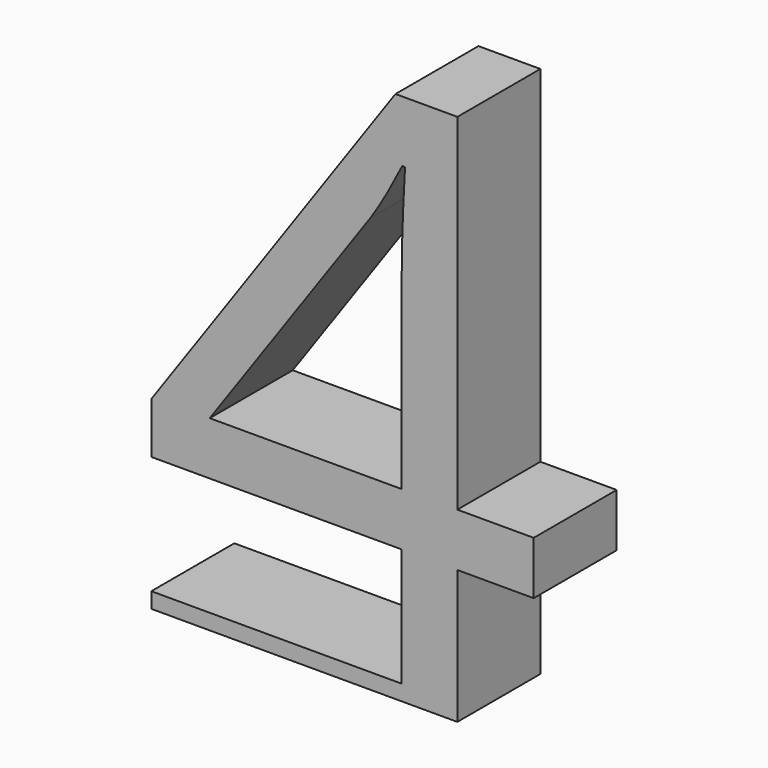
from build123d import *

# Parameters (mm, degrees)
F0_TEXT_SIZE  = 138.8888888889
F1_DEPTH      = 10
F1_DEPTH_BACK = 10
F2_W          = 59.0060763889
F2_H          = 20
F3_DEPTH      = 3


# Not quite as in the source:
# - Text() gives the source's letters only with a copy of the font that has no kerning and outlines rounded to 1/6400 em; it was checked with that copy


with BuildPart() as f1:
    # F0 (on Front) → F1 (new body, two sides)
    with BuildSketch(Plane.XZ) as f1_sk:
        with Locations((-42.8168402778, 0)):
            Text('4', F0_TEXT_SIZE, font='Open Sans', text_align=(TextAlign.LEFT, TextAlign.BOTTOM))
    extrude(amount=F1_DEPTH)
    extrude(f1_sk.sketch, amount=-F1_DEPTH_BACK)

    # F2 (on Top) → F3 (join)
    with BuildSketch(Plane.XY):
        with Locations((-10.4058159722, 0)):
            Rectangle(F2_W, F2_H)
    extrude(amount=-F3_DEPTH)


solid = f1.part
